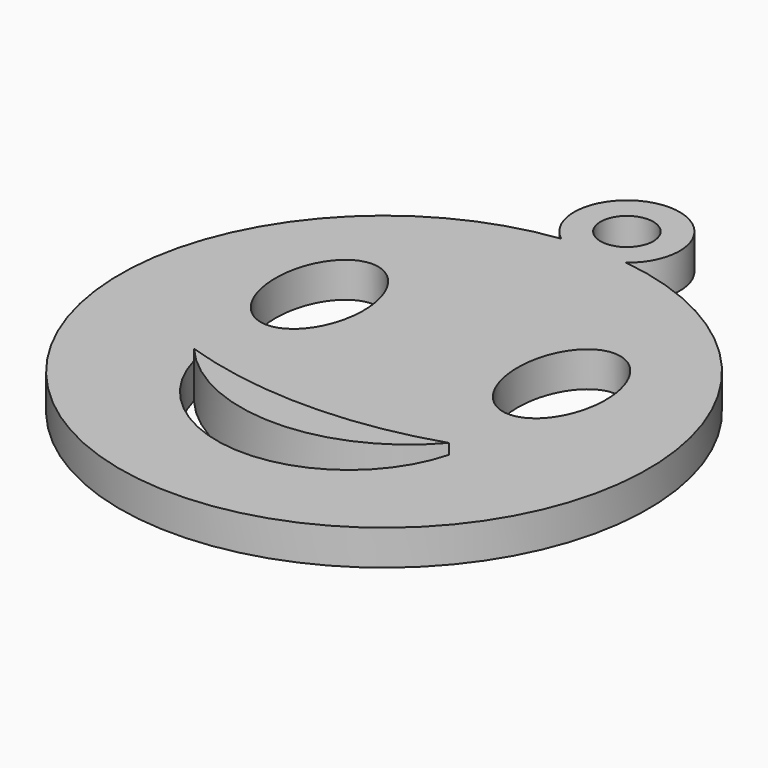
from build123d import *

# Parameters (mm, degrees)
F0_R          = 30
F1_DEPTH      = 4
F3_DEPTH      = 15.7
F5_DEPTH      = 14.1
F7_DEPTH      = 1.2
F7_DEPTH_BACK = 4.1
F8_R          = 6
F8_R_2        = 3
F9_DEPTH      = 4


# Not quite as in the source:
# - a feature names something its author has since deleted; it is built from what else it names


with BuildPart() as f1:
    # F0 (on Top) → F1 (new body)
    with BuildSketch(Plane.XY):
        Circle(F0_R)
        with BuildLine():
            ThreePointArc((18.5144313724, -15.5611746563), (-0.2600227829, -23.7984225598), (-18.8815741249, -15.2211148546))
            Line((-18.8815741249, -15.2211148546), (-16.6486222239, -13.9582220563))
            Line((-16.6486222239, -13.9582220563), (-14.4156703229, -12.695329258))
            ThreePointArc((-14.4156703229, -12.695329258), (-0.3525836389, -18.7968976895), (13.8984762541, -13.1482840248))
            Line((13.8984762541, -13.1482840248), (16.2064538132, -14.3547293405))
            Line((16.2064538132, -14.3547293405), (18.5144313724, -15.5611746563))
        make_face(mode=Mode.SUBTRACT)
        with BuildLine():
            add(Edge.make_bspline(
                [(-13.759398363, 15.5196315202), (-22.4196524008, 15.5196315202), (-18.0895253819, 4.2696315202), (-13.759398363, -6.9803684798), (-9.4292713441, 4.2696315202), (-5.0991443251, 15.5196315202), (-13.759398363, 15.5196315202)],
                knots=[0, 0, 0, 2.0943951024, 2.0943951024, 4.1887902048, 4.1887902048, 6.2831853072, 6.2831853072, 6.2831853072], degree=2, weights=[1, 0.5, 1, 0.5, 1, 0.5, 1]))
        make_face(mode=Mode.SUBTRACT)
        with BuildLine():
            add(Edge.make_bspline(
                [(13.759398363, 15.5196315202), (5.0991443251, 15.5196315202), (9.4292713441, 4.2696315202), (13.759398363, -6.9803684798), (18.0895253819, 4.2696315202), (22.4196524008, 15.5196315202), (13.759398363, 15.5196315202)],
                knots=[0, 0, 0, 2.0943951024, 2.0943951024, 4.1887902048, 4.1887902048, 6.2831853072, 6.2831853072, 6.2831853072], degree=2, weights=[1, 0.5, 1, 0.5, 1, 0.5, 1]))
        make_face(mode=Mode.SUBTRACT)
        with BuildLine():
            add(Edge.make_bspline(
                [(13.759398363, 15.5196315202), (5.0991443251, 15.5196315202), (9.4292713441, 4.2696315202), (13.759398363, -6.9803684798), (18.0895253819, 4.2696315202), (22.4196524008, 15.5196315202), (13.759398363, 15.5196315202)],
                knots=[0, 0, 0, 2.0943951024, 2.0943951024, 4.1887902048, 4.1887902048, 6.2831853072, 6.2831853072, 6.2831853072], degree=2, weights=[1, 0.5, 1, 0.5, 1, 0.5, 1]))
        make_face()
        with BuildLine():
            add(Edge.make_bspline(
                [(-13.759398363, 15.5196315202), (-22.4196524008, 15.5196315202), (-18.0895253819, 4.2696315202), (-13.759398363, -6.9803684798), (-9.4292713441, 4.2696315202), (-5.0991443251, 15.5196315202), (-13.759398363, 15.5196315202)],
                knots=[0, 0, 0, 2.0943951024, 2.0943951024, 4.1887902048, 4.1887902048, 6.2831853072, 6.2831853072, 6.2831853072], degree=2, weights=[1, 0.5, 1, 0.5, 1, 0.5, 1]))
        make_face()
        with BuildLine():
            Line((-14.4156703229, -12.695329258), (-16.6486222239, -13.9582220563))
            ThreePointArc((-16.6486222239, -13.9582220563), (-0.3057099111, -21.168664653), (16.2064538132, -14.3547293405))
            Line((16.2064538132, -14.3547293405), (13.8984762541, -13.1482840248))
            ThreePointArc((13.8984762541, -13.1482840248), (-0.3525836389, -18.7968976895), (-14.4156703229, -12.695329258))
        make_face()
        with BuildLine():
            Line((-16.6486222239, -13.9582220563), (-18.8815741249, -15.2211148546))
            ThreePointArc((-18.8815741249, -15.2211148546), (-0.2600227829, -23.7984225598), (18.5144313724, -15.5611746563))
            Line((18.5144313724, -15.5611746563), (16.2064538132, -14.3547293405))
            ThreePointArc((16.2064538132, -14.3547293405), (-0.3057099111, -21.168664653), (-16.6486222239, -13.9582220563))
        make_face()
    extrude(amount=F1_DEPTH)

    # F2 (on face) → F3 (cut)
    with BuildSketch(Plane.XY.offset(4)):
        with BuildLine():
            ThreePointArc((14.4841292455, -8.9), (0, -11.2132519808), (-14.4841292455, -8.9))
            ThreePointArc((-14.4841292455, -8.9), (0, -20), (14.4841292455, -8.9))
        make_face()
    extrude(amount=-F3_DEPTH, mode=Mode.SUBTRACT)

    # F0 (on Top) → F5 (cut)
    with BuildSketch(Plane.XY):
        with BuildLine():
            add(Edge.make_bspline(
                [(-13.759398363, 15.5196315202), (-22.4196524008, 15.5196315202), (-18.0895253819, 4.2696315202), (-13.759398363, -6.9803684798), (-9.4292713441, 4.2696315202), (-5.0991443251, 15.5196315202), (-13.759398363, 15.5196315202)],
                knots=[0, 0, 0, 2.0943951024, 2.0943951024, 4.1887902048, 4.1887902048, 6.2831853072, 6.2831853072, 6.2831853072], degree=2, weights=[1, 0.5, 1, 0.5, 1, 0.5, 1]))
        make_face()
        with BuildLine():
            add(Edge.make_bspline(
                [(13.759398363, 15.5196315202), (5.0991443251, 15.5196315202), (9.4292713441, 4.2696315202), (13.759398363, -6.9803684798), (18.0895253819, 4.2696315202), (22.4196524008, 15.5196315202), (13.759398363, 15.5196315202)],
                knots=[0, 0, 0, 2.0943951024, 2.0943951024, 4.1887902048, 4.1887902048, 6.2831853072, 6.2831853072, 6.2831853072], degree=2, weights=[1, 0.5, 1, 0.5, 1, 0.5, 1]))
        make_face()
    extrude(amount=F5_DEPTH, mode=Mode.SUBTRACT)

    # F6 (on face) → F7 (join, two sides)
    with BuildSketch(Plane.XY.offset(4)) as f7_sk:
        with BuildLine():
            ThreePointArc((14.4841292455, -8.9), (0, -11.2132519808), (-14.4841292455, -8.9))
            ThreePointArc((-14.4841292455, -8.9), (0, -15.581886089), (14.4841292455, -8.9))
        make_face()
    extrude(amount=F7_DEPTH)
    extrude(f7_sk.sketch, amount=-F7_DEPTH_BACK)

    # F8 (on face) → F9 (join)
    with BuildSketch(Plane.XY.offset(4)):
        with Locations((0, 34.5)):
            Circle(F8_R)
        with Locations((0, 34.5)):
            Circle(F8_R_2, mode=Mode.SUBTRACT)
    extrude(amount=-F9_DEPTH)


solid = f1.part
